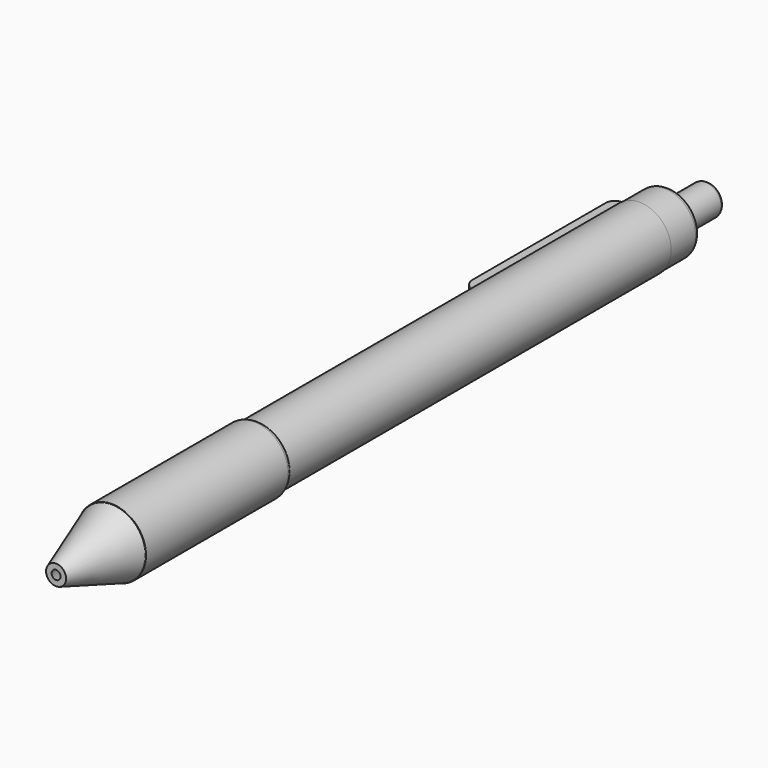
from build123d import *

# Parameters (mm, degrees)
F0_R      = 4.4185747542
F1_DEPTH  = 33.274
F2_R      = 4.3520524893
F3_DEPTH  = 5.08
F4_R      = 2.2018395717
F5_DEPTH  = 6.858
F6_R      = 4.7683130079
F6_R_2    = 4.4185747542
F7_DEPTH  = 25.4
F12_W     = 26.4561073855
F12_H     = 1.6188730951
F13_DEPTH = 1.6002
F17_R     = 0.0508
F18_R     = 0.508
F19_R     = 0.762
F20_R     = 1.27
F21_SIZE  = 1.27
F22_R     = 0.508
F23_R     = 0.127
F24_R     = 1.8805178093


# Not quite as in the source:
# - a fillet or chamfer that OpenCascade refuses, or shapes differently, is made with other operations: its cross-section is extruded or revolved along the edge and cut away or added
# - the program builds the solid bodies; features that only make, move or delete a surface that nothing else refers to are left out


with BuildPart() as f1:
    # F0 (on Front) → F1 (new body, symmetric)
    with BuildSketch(Plane.XZ):
        Circle(F0_R)
    extrude(amount=F1_DEPTH, both=True)

    # F2 (on face) → F3 (join)
    with BuildSketch(Plane(origin=(0, 33.274, 0), x_dir=(-1, 0, 0), z_dir=(0, 1, 0))):
        Circle(F2_R)
    extrude(amount=F3_DEPTH)

    # F4 (on face) → F5 (join)
    with BuildSketch(Plane(origin=(0, 38.354, 0), x_dir=(-1, 0, 0), z_dir=(0, 1, 0))):
        Circle(F4_R)
    extrude(amount=F5_DEPTH)

    # F18
    f18_edges = [f1.edges().sort_by_distance(p)[0] for p in [
        (2.20184, 45.212, 0),
    ]]
    fillet(f18_edges, radius=F18_R)

    # F19
    f19_edges = [f1.edges().sort_by_distance(p)[0] for p in [
        (4.352052, 38.354, 0),
    ]]
    fillet(f19_edges, radius=F19_R)


with BuildPart() as f7:
    # F6 (on face) → F7 (new body)
    with BuildSketch(Plane.XZ.offset(33.274)):
        Circle(F6_R)
        Circle(F6_R_2, mode=Mode.SUBTRACT)
    extrude(amount=F7_DEPTH)

    # F16: fillet of radius 0.762 on 1 edges, made by hand

    # F16_s1 → F16_t2 (revolve, cut)
    with BuildSketch(Plane.XY):
        with BuildLine():
            ThreePointArc((4.7684630079, -33.9147646456), (4.6753183658, -33.5496940905), (4.4186558946, -33.2738738404))
            Line((4.4186558946, -33.2738738404), (4.4268997523, -33.2610560243))
            ThreePointArc((4.4268997523, -33.2610560243), (4.5934844512, -33.25876), (4.7683130079, -33.25876))
            Line((4.7683130079, -33.25876), (4.7835530079, -33.274))
            ThreePointArc((4.7835530079, -33.274), (4.7835530079, -33.5943823228), (4.7837030079, -33.9147646456))
            Line((4.7837030079, -33.9147646456), (4.7684630079, -33.9147646456))
        make_face()
    revolve(axis=Axis((0, -33.274, 0), (0, -1, 0)), mode=Mode.SUBTRACT)

    # F17
    f17_edges = [f7.edges().sort_by_distance(p)[0] for p in [
        (-4.768313, -58.674, 0),
    ]]
    fillet(f17_edges, radius=F17_R)


with BuildPart() as f13:
    # F12 (on offset) → F13 (new body)
    with BuildSketch(Plane.YZ.offset(-5.6134)):
        with Locations((24.4508138858, -0.1013565925)):
            Rectangle(F12_W, F12_H)
    extrude(amount=-F13_DEPTH)

    # F20
    f20_edges = [f13.edges().sort_by_distance(p)[0] for p in [
        (-7.2136, 37.678868, -0.101357),
    ]]
    fillet(f20_edges, radius=F20_R)

    # F21
    f21_edges = [f13.edges().sort_by_distance(p)[0] for p in [
        (-7.2136, 11.22276, -0.101357),
    ]]
    chamfer(f21_edges, length=F21_SIZE)

    # F22
    f22_edges = [f13.edges().sort_by_distance(p)[0] for p in [
        (-5.9436, 11.22276, -0.101357),
    ]]
    fillet(f22_edges, radius=F22_R)

    # F23
    f23_edges = [f13.edges().sort_by_distance(p)[0] for p in [
        (-5.6134, 11.22276, -0.101357),
    ]]
    fillet(f23_edges, radius=F23_R)

    # F24
    f24_edges = [f13.edges().sort_by_distance(p)[0] for p in [
        (-7.2136, 12.49276, -0.101357),
    ]]
    fillet(f24_edges, radius=F24_R)


with BuildPart() as f15:
    # F14 (on Top) → F15 (revolve)
    with BuildSketch(Plane.XY):
        Polygon((1.394969644, -68.3624893427), (4.7210464254, -58.6740672588), (0.6249820581, -68.3624893427), align=None)
    revolve(axis=Axis((0, -58.674, 0), (0, -1, 0)))


solid = Compound([f1.part, f7.part, f13.part, f15.part])
